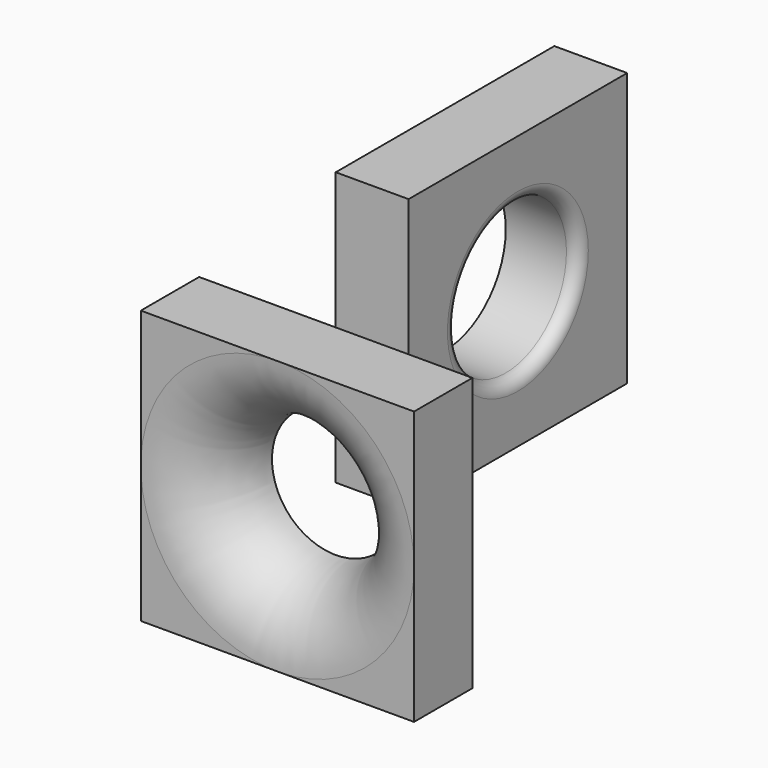
from build123d import *

# Parameters (mm, degrees)
F0_W     = 45
F0_H     = 45
F0_R     = 10.5
F1_DEPTH = 12
F2_R     = 11.99999
F3_W     = 45
F3_H     = 45
F3_R     = 12.5
F4_DEPTH = 12
F5_R     = 2


# Not quite as in the source:
# - a fillet or chamfer is up to 0.001 mm smaller than in the source, because OpenCascade refuses the exact size


with BuildPart() as f1:
    # F0 (on Front) → F1 (new body)
    with BuildSketch(Plane.XZ):
        Rectangle(F0_W, F0_H)
        Circle(F0_R, mode=Mode.SUBTRACT)
    extrude(amount=F1_DEPTH)

    # F2 (radius 12 in the source; OpenCascade refuses exactly that, so slightly less here)
    f2_edges = [f1.edges().sort_by_distance(p)[0] for p in [
        (-10.5, -12, 0),
    ]]
    fillet(f2_edges, radius=F2_R)


with BuildPart() as f4:
    # F3 (on Right) → F4 (new body)
    with BuildSketch(Plane.YZ):
        with Locations((22.5, 22.5)):
            Rectangle(F3_W, F3_H)
        with Locations((22.5, 22.5)):
            Circle(F3_R, mode=Mode.SUBTRACT)
    extrude(amount=F4_DEPTH)

    # F5
    f5_edges = [f4.edges().sort_by_distance(p)[0] for p in [
        (12, 10, 22.5),
    ]]
    fillet(f5_edges, radius=F5_R)


solid = Compound([f1.part, f4.part])
